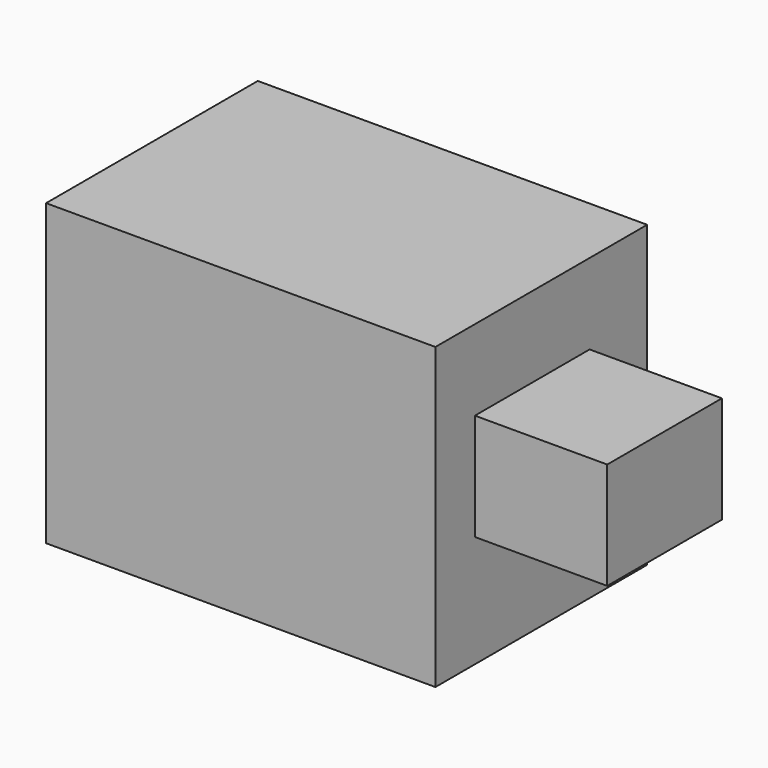
from build123d import *

# Parameters (mm, degrees)
F0_W     = 37.3699069023
F0_H     = 28.7381336093
F1_DEPTH = 25.4
F4_W     = 13.7605443597
F4_H     = 10.2546699345
F5_DEPTH = 12.7


# Not quite as in the source:
# - the program builds the solid bodies; features that only make, move or delete a surface that nothing else refers to are left out


with BuildPart() as f1:
    # F0 (on Front) → F1 (new body)
    with BuildSketch(Plane.XZ):
        with Locations((18.6849534512, -14.3690668046)):
            Rectangle(F0_W, F0_H)
    extrude(amount=F1_DEPTH)

    # F4 (on face) → F5 (join)
    with BuildSketch(Plane.YZ.offset(37.3699069023)):
        with Locations((-13.7830860913, -12.8563437611)):
            Rectangle(F4_W, F4_H)
    extrude(amount=F5_DEPTH)


solid = f1.part
